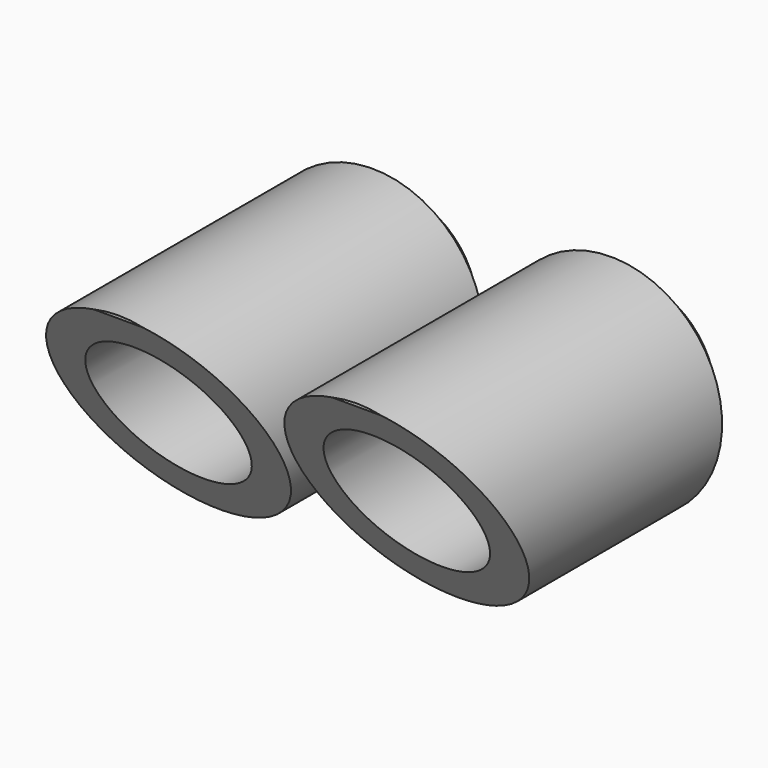
from build123d import *

# Parameters (mm, degrees)
F0_R          = 44.45
F1_DEPTH      = 127
F2_R          = 31.75
F3_DEPTH      = 12.7
F4_R          = 30.226
F5_DEPTH      = 139.701
F7_DEPTH      = 82.76927268
F7_DEPTH_BACK = 101.38272732


with BuildPart() as f1:
    # F0 (on Front) → F1 (new body)
    with BuildSketch(Plane.XZ):
        with Locations((-38.31827268, 0)):
            Circle(F0_R)
    extrude(amount=F1_DEPTH)


with BuildPart() as f1b:
    # F0 (on Front) → F1, piece 2 (new body)
    with BuildSketch(Plane.XZ):
        with BuildLine():
            ThreePointArc((101.38172732, 0), (56.93172732, 44.45), (12.48172732, 0))
            ThreePointArc((12.48172732, 0), (56.93172732, -44.45), (101.38172732, 0))
        make_face()
    extrude(amount=F1_DEPTH)


with BuildPart() as f3:
    # F2 (on face) → F3 (new body)
    with BuildSketch(Plane(origin=(0, 0, 0), x_dir=(-1, 0, 0), z_dir=(0, 1, 0))):
        with Locations((38.31827268, 0)):
            Circle(F2_R)
    extrude(amount=F3_DEPTH)


with BuildPart() as f3b:
    # F2 (on face) → F3, piece 2 (new body)
    with BuildSketch(Plane(origin=(0, 0, 0), x_dir=(-1, 0, 0), z_dir=(0, 1, 0))):
        with Locations((-56.93172732, 0)):
            Circle(F2_R)
    extrude(amount=F3_DEPTH)


with BuildPart() as f5_tool:
    # F4 (on face) → F5 (new body, through all)
    with BuildSketch(Plane(origin=(0, 12.7, 0), x_dir=(-1, 0, 0), z_dir=(0, 1, 0))):
        with Locations((-56.93172732, 0)):
            Circle(F4_R)
        with Locations((38.31827268, 0)):
            Circle(F4_R)
    extrude(amount=-F5_DEPTH)


with BuildPart() as f1_1:
    add(f1.part)

    # F5: cut by f5_tool
    add(f5_tool.part, mode=Mode.SUBTRACT)


with BuildPart() as f1b_1:
    add(f1b.part)

    # F5: cut by f5_tool
    add(f5_tool.part, mode=Mode.SUBTRACT)


with BuildPart() as f3_1:
    add(f3.part)

    # F5: cut by f5_tool
    add(f5_tool.part, mode=Mode.SUBTRACT)


with BuildPart() as f3b_1:
    add(f3b.part)

    # F5: cut by f5_tool
    add(f5_tool.part, mode=Mode.SUBTRACT)


with BuildPart() as f7_tool:
    # F6 (on Right) → F7 (new body, two sides)
    with BuildSketch(Plane.YZ) as f7_sk:
        Polygon((-59.1113475329, -74.2536739212), (-133.0174654722, 53.7554773399), (-133.0174654722, -74.2536739212), align=None)
    extrude(amount=-F7_DEPTH)
    extrude(f7_sk.sketch, amount=F7_DEPTH_BACK)


with BuildPart() as f1_2:
    add(f1_1.part)

    # F7: cut by f7_tool
    add(f7_tool.part, mode=Mode.SUBTRACT)


with BuildPart() as f1b_2:
    add(f1b_1.part)

    # F7: cut by f7_tool
    add(f7_tool.part, mode=Mode.SUBTRACT)


solid = Compound([f3_1.part, f3b_1.part, f1_2.part, f1b_2.part])
